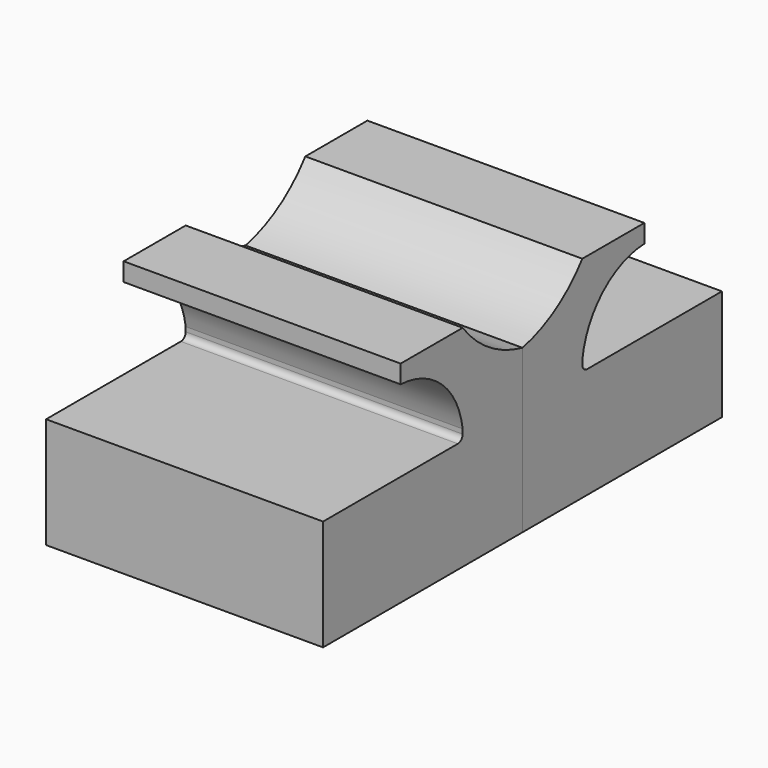
from build123d import *

# Parameters (mm, degrees)
F1_DEPTH = 10


# Not quite as in the source:
# - a pattern or mirror of a feature is missing from the dataset's text; its kind, count and spacing are read off the source's solid


with BuildPart() as f1:
    # F0 (on Right) → F1 (new body)
    with BuildSketch(Plane.YZ):
        with BuildLine():
            Line((5.5, 2.3115177173), (2.7, 2.3115177173))
            ThreePointArc((2.7, 2.3115177173), (1.5050999961, 1.2033549585), (0, 0.5784671916))
            Line((0, 0.5784671916), (0, -5.2862326842))
            Line((0, -5.2862326842), (9, -5.2862326842))
            Line((9, -5.2862326842), (9, -1.2862326842))
            Line((9, -1.2862326842), (2.9180552616, -1.2862326842))
            ThreePointArc((2.9180552616, -1.2862326842), (2.7638669074, -1.2223657768), (2.7, -1.0681774227))
            Line((2.7, -1.0681774227), (2.7, -0.9035626068))
            ThreePointArc((2.7, -0.9035626068), (3.6332473174, 0.8854712641), (5.5, 1.6515177173))
            Line((5.5, 1.6515177173), (5.5, 2.3115177173))
        make_face()
    extrude(amount=F1_DEPTH)


with BuildPart() as f1_copies_1:
    # F1_copies: instance of F1
    add(f1.part.mirror(Plane(origin=(0, 0, 0), x_dir=(0, 0, -1), z_dir=(0, -1, 0))))


solid = Compound([f1.part, f1_copies_1.part])
